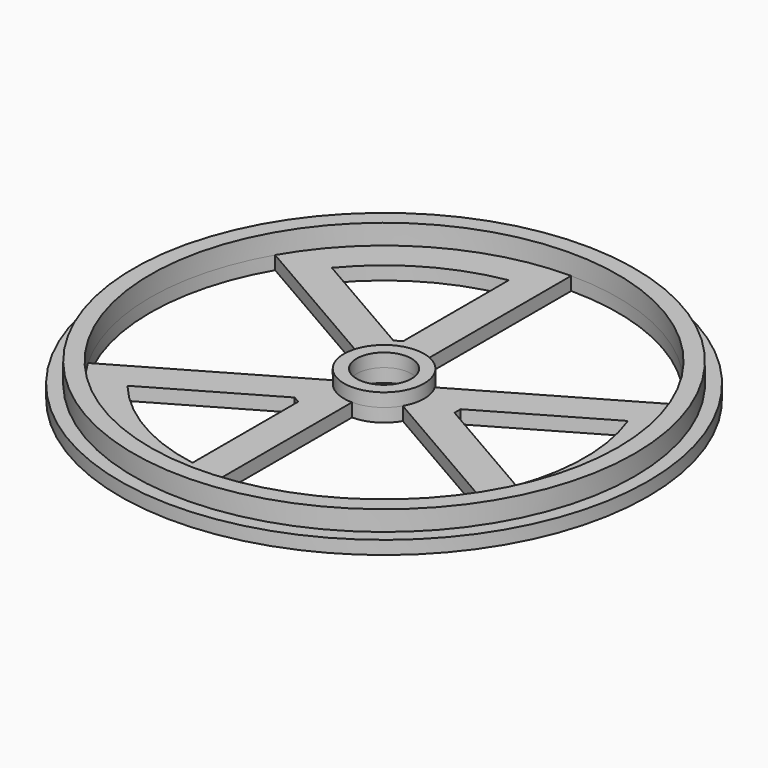
from build123d import *
from build123d import SkipClean  # not in build123d's __all__

# Parameters (mm, degrees)
F0_R      = 39.5
F1_DEPTH  = 2
F2_R      = 37.5
F2_R_2    = 35
F3_DEPTH  = 3
F4_R      = 4.1
F5_DEPTH  = 25
F6_R      = 6
F6_R_2    = 4.1
F7_DEPTH  = 2
F9_DEPTH  = 25
F11_DEPTH = 25


# Not quite as in the source:
# - after a boolean that leaves OpenCascade's solid faulty, fix() repairs it


with BuildPart() as f1:
    # F0 (on Top) → F1 (new body)
    with BuildSketch(Plane.XY):
        Circle(F0_R)
    extrude(amount=F1_DEPTH)

    # F2 (on face) → F3 (join)
    with BuildSketch(Plane.XY.offset(2)):
        Circle(F2_R)
        Circle(F2_R_2, mode=Mode.SUBTRACT)
    extrude(amount=F3_DEPTH)

    # F4 (on face) → F5 (cut)
    with BuildSketch(Plane.XY.offset(2)):
        Circle(F4_R)
    extrude(amount=-F5_DEPTH, mode=Mode.SUBTRACT)

    # F6 (on face) → F7 (join)
    with BuildSketch(Plane.XY.offset(2)):
        Circle(F6_R)
        Circle(F6_R_2, mode=Mode.SUBTRACT)
    extrude(amount=F7_DEPTH)

    # F8 (on face) → F9 (cut)
    with BuildSketch(Plane.XY.offset(2)):
        with BuildLine():
            Line((30.3108891325, 17.5), (0, 35))
            Line((0, 35), (0, 6))
            ThreePointArc((0, 6), (3, 5.1961524227), (5.1961524227, 3))
            Line((5.1961524227, 3), (30.3108891325, 17.5))
        make_face()
        with BuildLine():
            Line((0, -35), (30.3108891325, -17.5))
            Line((30.3108891325, -17.5), (5.1961524227, -3))
            ThreePointArc((5.1961524227, -3), (3, -5.1961524227), (0, -6))
            Line((0, -6), (0, -35))
        make_face()
        with BuildLine():
            ThreePointArc((30.3108891325, 17.5), (17.5, 30.3108891325), (0, 35))
            Line((0, 35), (30.3108891325, 17.5))
        make_face()
        with BuildLine():
            ThreePointArc((0, -35), (17.5, -30.3108891325), (30.3108891325, -17.5))
            Line((30.3108891325, -17.5), (0, -35))
        make_face()
        with BuildLine():
            Line((-5.1961524227, 3), (-30.3108891325, 17.5))
            Line((-30.3108891325, 17.5), (-30.3108891325, -17.5))
            Line((-30.3108891325, -17.5), (-5.1961524227, -3))
            ThreePointArc((-5.1961524227, -3), (-6, 0), (-5.1961524227, 3))
        make_face()
        with BuildLine():
            Line((-30.3108891325, -17.5), (-30.3108891325, 17.5))
            ThreePointArc((-30.3108891325, 17.5), (-35, 0), (-30.3108891325, -17.5))
        make_face()
    with SkipClean():  # cleaning this boolean's faces spoils the solid; the shape is the same uncleaned
        extrude(amount=-F9_DEPTH, mode=Mode.SUBTRACT)

    # F10 (on face) → F11 (cut)
    with BuildSketch(Plane.XY.offset(2)):
        with BuildLine():
            Line((-5, 9.7979589711), (-5, 29.5803989155))
            ThreePointArc((-5, 29.5803989155), (-15, 25.9807621135), (-23.1173769149, 19.1203264767))
            Line((-23.1173769149, 19.1203264767), (-5.9852813742, 9.2291065045))
            ThreePointArc((-5.9852813742, 9.2291065045), (-5.5, 9.5262794416), (-5, 9.7979589711))
        make_face()
        with BuildLine():
            ThreePointArc((10.9852813742, 0.5688524666), (11, 0), (10.9852813742, -0.5688524666))
            Line((10.9852813742, -0.5688524666), (28.1173769149, -10.4600724388))
            ThreePointArc((28.1173769149, -10.4600724388), (30, 0), (28.1173769149, 10.4600724388))
            Line((28.1173769149, 10.4600724388), (10.9852813742, 0.5688524666))
        make_face()
        with BuildLine():
            ThreePointArc((-5, -9.7979589711), (-5.5, -9.5262794416), (-5.9852813742, -9.2291065045))
            Line((-5.9852813742, -9.2291065045), (-23.1173769149, -19.1203264767))
            ThreePointArc((-23.1173769149, -19.1203264767), (-15, -25.9807621135), (-5, -29.5803989155))
            Line((-5, -29.5803989155), (-5, -9.7979589711))
        make_face()
    extrude(amount=-F11_DEPTH, mode=Mode.SUBTRACT)

    add(f1.part.fix(), mode=Mode.REPLACE)


solid = f1.part
